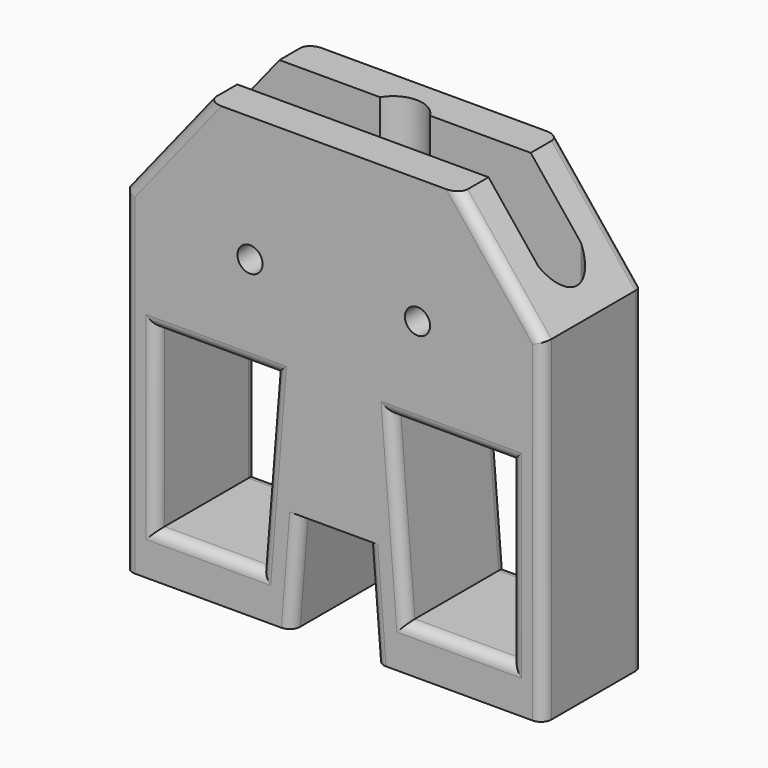
from build123d import *

# Parameters (mm, degrees)
F1_DEPTH  = 9.525
F3_DEPTH  = 30.48
F4_R      = 3.556
F5_DEPTH  = 36.195
F7_DEPTH  = 12.7
F8_R      = 1.5875
F9_R      = 1.905
F10_DEPTH = 19.05


# Not quite as in the source:
# - a feature names something its author has since deleted; it is built from what else it names


with BuildPart() as f1:
    # F0 (on Front) → F1 (new body, symmetric)
    with BuildSketch(Plane.XZ):
        Polygon((-31.75, 50.8), (-31.75, 0), (-6.35, 0), (-5.08, 15.875), (0, 15.875), (0, 66.675), (-19.05, 66.675), align=None)
        Polygon((19.05, 66.675), (0, 66.675), (0, 15.875), (5.08, 15.875), (6.35, 0), (31.75, 0), (31.75, 50.8), align=None)
    extrude(amount=F1_DEPTH, both=True)

    # F2 (on face) → F3 (cut)
    with BuildSketch(Plane.XY.offset(66.675)):
        with BuildLine():
            Line((26.67, -4.0005), (26.67, 4.0005))
            Line((26.67, 4.0005), (3.7759814618, 4.0005))
            ThreePointArc((3.7759814618, 4.0005), (0, 6.1595), (-3.7759814618, 4.0005))
            Line((-3.7759814618, 4.0005), (-26.67, 4.0005))
            Line((-26.67, 4.0005), (-26.67, -4.0005))
            Line((-26.67, -4.0005), (26.67, -4.0005))
        make_face()
        with BuildLine():
            ThreePointArc((26.67, -4.0005), (29.2644515955, 0), (26.67, 4.0005))
            Line((26.67, 4.0005), (26.67, -4.0005))
        make_face()
        with BuildLine():
            ThreePointArc((-26.67, 4.0005), (-29.2644515955, 0), (-26.67, -4.0005))
            Line((-26.67, -4.0005), (-26.67, 4.0005))
        make_face()
    extrude(amount=-F3_DEPTH, mode=Mode.SUBTRACT)

    # F4 (on Top) → F5 (cut, through all)
    with BuildSketch(Plane.XY):
        Circle(F4_R)
    extrude(amount=F5_DEPTH, mode=Mode.SUBTRACT)

    # F6 (on Front) → F7 (cut, symmetric)
    with BuildSketch(Plane.XZ):
        Polygon((-8.89, 33.5468458159), (-26.9126990667, 33.5468458159), (-26.9126990667, 6.7006074823), (-11.0376990667, 6.7006074823), align=None)
        Polygon((8.89, 33.5468458159), (11.0376990667, 6.7006074823), (26.9126990667, 6.7006074823), (26.9126990667, 33.5468458159), align=None)
    extrude(amount=F7_DEPTH, both=True, mode=Mode.SUBTRACT)

    # F8
    f8_edges = [f1.edges().sort_by_distance(p)[0] for p in [
        (31.75, 9.525, 25.4),
        (25.4, 9.525, 58.7375),
        (31.75, -9.525, 25.4),
        (25.4, -9.525, 58.7375),
        (5.715, 9.525, 7.9375),
        (5.715, -9.525, 7.9375),
        (-5.715, -9.525, 7.9375),
        (-5.715, 9.525, 7.9375),
        (-31.75, 9.525, 25.4),
        (-31.75, -9.525, 25.4),
        (-25.4, 9.525, 58.7375),
        (-25.4, -9.525, 58.7375),
        (-17.90135, 9.525, 33.546846),
        (-26.912699, 9.525, 20.123727),
        (-18.975199, 9.525, 6.700607),
        (-9.96385, 9.525, 20.123727),
        (9.96385, 9.525, 20.123727),
        (18.975199, 9.525, 6.700607),
        (26.912699, 9.525, 20.123727),
        (17.90135, 9.525, 33.546846),
        (-17.90135, -9.525, 33.546846),
        (-26.912699, -9.525, 20.123727),
        (-18.975199, -9.525, 6.700607),
        (-9.96385, -9.525, 20.123727),
        (9.96385, -9.525, 20.123727),
        (18.975199, -9.525, 6.700607),
        (26.912699, -9.525, 20.123727),
        (17.90135, -9.525, 33.546846),
    ]]
    fillet(f8_edges, radius=F8_R)

    # F9 (on face) → F10 (cut, through all)
    with BuildSketch(Plane(origin=(0, 9.525, 0), x_dir=(-1, 0, 0), z_dir=(0, 1, 0))):
        with Locations((-12.7, 47.625)):
            Circle(F9_R)
        with Locations((12.7, 47.625)):
            Circle(F9_R)
    extrude(amount=-F10_DEPTH, mode=Mode.SUBTRACT)


solid = f1.part
